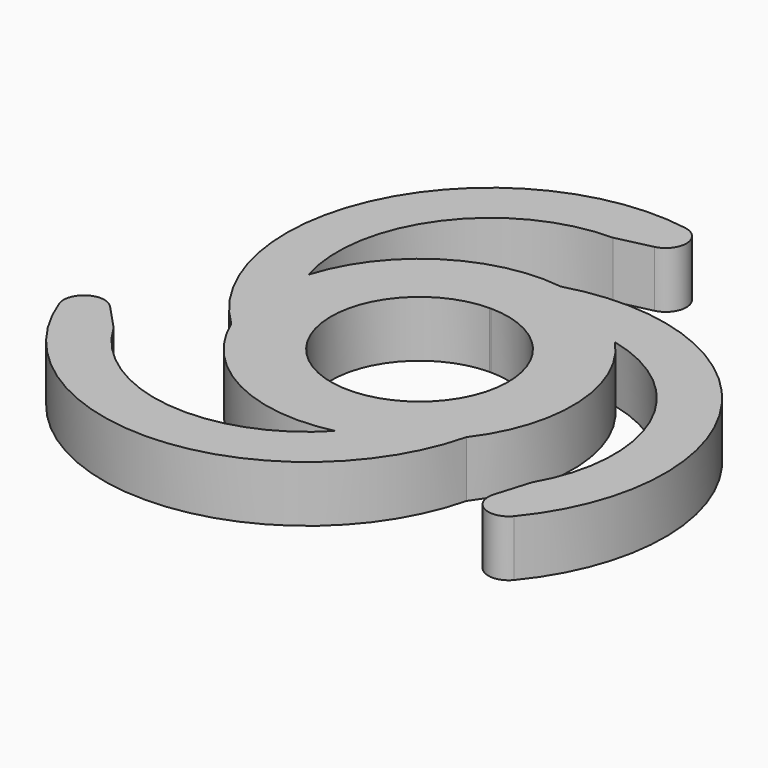
from build123d import *

# Parameters (mm, degrees)
F1_DEPTH = 7
F2_R     = 2.54


# Not quite as in the source:
# - a feature names something its author has since deleted; it is built from what else it names


with BuildPart() as f1:
    # F0 (on Top) → F1 (new body)
    with BuildSketch(Plane.XY):
        with BuildLine():
            ThreePointArc((12.7, 33.0220452561), (-20.3035705189, 26.2868814104), (-17.6006612279, -7.2882936508))
            ThreePointArc((-17.6006612279, -7.2882936508), (-8.6968003579, -16.9489870947), (4.3435297347, -18.5482141848))
            ThreePointArc((4.3435297347, -18.5482141848), (-11.7341390993, -24.436637764), (-26.0457140188, -15.0375))
            Line((-26.0457140188, -15.0375), (-34.9479300767, -5.5125))
            ThreePointArc((-34.9479300767, -5.5125), (-12.6133218282, -30.7268485621), (15.1121780658, -11.5984729214))
            ThreePointArc((15.1121780658, -11.5984729214), (19.0266535713, 0.9428435058), (13.8914598115, 13.0357141848))
            ThreePointArc((13.8914598115, 13.0357141848), (27.0298186363, 2.0562563305), (26.0457140188, -15.0375))
            Line((26.0457140188, -15.0375), (22.2479300767, -27.5095452561))
            ThreePointArc((22.2479300767, -27.5095452561), (32.9168923471, 4.4399671517), (2.4884831621, 18.8867665722))
            ThreePointArc((2.4884831621, 18.8867665722), (-10.3298532135, 16.0061435889), (-18.2349895462, 5.5125))
            ThreePointArc((-18.2349895462, 5.5125), (-15.295679537, 22.3803814335), (0, 30.075))
            Line((0, 30.075), (12.7, 33.0220452561))
        make_face()
        with BuildLine():
            ThreePointArc((0.0913914699, 11.0246211998), (7.8280973408, 7.7634732577), (11.025, 0))
            ThreePointArc((11.025, 0), (10.6610677893, -2.8093163923), (9.5932977611, -5.4331632653))
            ThreePointArc((9.5932977611, -5.4331632653), (9.5479300767, -5.5125), (9.5019062912, -5.5914579345))
            ThreePointArc((9.5019062912, -5.5914579345), (0, -11.025), (-9.5019062912, -5.5914579345))
            ThreePointArc((-9.5019062912, -5.5914579345), (-9.5479300767, -5.5125), (-9.5932977611, -5.4331632653))
            ThreePointArc((-9.5932977611, -5.4331632653), (-9.5479300767, 5.5125), (-0.0913914699, 11.0246211998))
            ThreePointArc((-0.0913914699, 11.0246211998), (0, 11.025), (0.0913914699, 11.0246211998))
        make_face(mode=Mode.SUBTRACT)
    extrude(amount=F1_DEPTH)

    # F2
    f2_edges = [f1.edges().sort_by_distance(p)[0] for p in [
        (12.7, 33.022045, 3.5),
        (22.24793, -27.509545, 3.5),
        (-34.94793, -5.5125, 3.5),
    ]]
    fillet(f2_edges, radius=F2_R)


solid = f1.part
